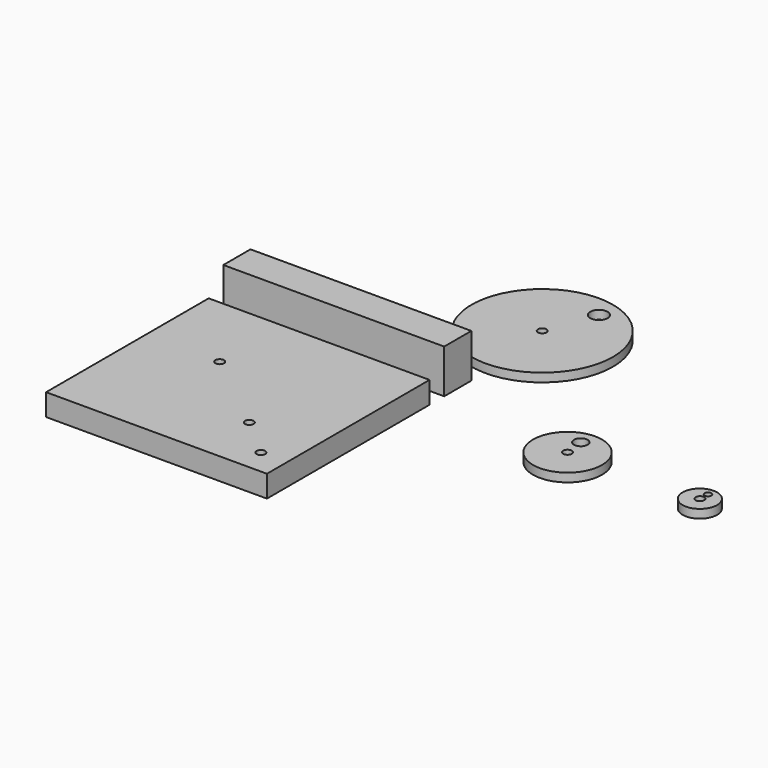
from build123d import *

# Parameters (mm, degrees)
F1_R             = 10
F1_R_2           = 1.9724824491
F2_DEPTH         = 2.5
F1_R_3           = 5
F1_R_4           = 0.9790800152
F0_R             = 20.5
F0_R_2           = 2.5126354118
F3_W             = 64.0254840255
F3_H             = 58.9180318639
F4_DEPTH         = 6.35
F3_H_2           = 9.8366048187
F5_DEPTH         = 6.35
F6_D             = 2.5
F8_D             = 2.5
F8_COPIES_COUNT  = 2
F8_COPIES_PITCH  = 30.5
F8_COPIES1_COUNT = 2
F8_COPIES1_PITCH = 45.489759
F10_D            = 2.5
F10_2_D          = 2.5


# Not quite as in the source:
# - a feature of the source that left no trace in its solid (it failed there, or was rolled back) is left out
# - a pattern or mirror of a feature is missing from the dataset's text; its kind, count and spacing are read off the source's solid


with BuildPart() as f2:
    # F1 (on Top) → F2 (new body)
    with BuildSketch(Plane.XY):
        with Locations((-4.1198744439, 6.6673322581)):
            Circle(F1_R)
        with Locations((-4.8270216212, 12.3583702371)):
            Circle(F1_R_2, mode=Mode.SUBTRACT)
    extrude(amount=F2_DEPTH)

    # F10 (through all)
    with Locations(Plane(origin=(0, 0, 0), x_dir=(1, 0, 0), z_dir=(0, 0, -1))):
        with Locations((-4.1198744439, -6.6673322581), (33.4935821593, -7.599897217)):
            Hole(F10_D / 2)


with BuildPart() as f2b:
    # F1 (on Top) → F2, piece 2 (new body)
    with BuildSketch(Plane.XY):
        with Locations((33.4935821593, 7.599897217)):
            Circle(F1_R_3)
        with Locations((33.6022078991, 10.4110669345)):
            Circle(F1_R_4, mode=Mode.SUBTRACT)
    extrude(amount=F2_DEPTH)

    # F10#2 (through all)
    with Locations(Plane(origin=(0, 0, 0), x_dir=(1, 0, 0), z_dir=(0, 0, -1))):
        with Locations((-4.1198744439, -6.6673322581), (33.4935821593, -7.599897217)):
            Hole(F10_2_D / 2)


with BuildPart() as f2c:
    # F0 (on Top) → F2, piece 3 (new body)
    with BuildSketch(Plane.XY):
        with Locations((-45.774448663, 49.5653226972)):
            Circle(F0_R)
        with Locations((-40.6095050275, 63.6612325907)):
            Circle(F0_R_2, mode=Mode.SUBTRACT)
    extrude(amount=F2_DEPTH)

    # F6 (through all)
    with Locations(Plane(origin=(0, 0, 0), x_dir=(1, 0, 0), z_dir=(0, 0, -1))):
        with Locations((-45.774448663, -49.5653226972)):
            Hole(F6_D / 2)


with BuildPart() as f4:
    # F3 (on Top) → F4 (new body)
    with BuildSketch(Plane.XY):
        with Locations((-78.0650638044, -20.3869701363)):
            Rectangle(F3_W, F3_H)
    extrude(amount=F4_DEPTH)

    # F8 (through all)
    with Locations(Plane.XY.offset(6.35)):
        with Locations((-88.7101224427, -13.6320184063)):
            f8 = Hole(F8_D / 2)

    # F8_copies: F8 ×2
    with Locations(*[Vector(0.7808687891, -0.6246950729, 0) * (i * F8_COPIES_PITCH) for i in range(1, F8_COPIES_COUNT)]):
        add(f8, mode=Mode.SUBTRACT)

    # F8_copies1: F8 ×2
    with Locations(*[Vector(0.7714882729, -0.636243542, 0) * (i * F8_COPIES1_PITCH) for i in range(1, F8_COPIES1_COUNT)]):
        add(f8, mode=Mode.SUBTRACT)


with BuildPart() as f4b:
    # F3 (on Top) → F4, piece 2 (new body)
    with BuildSketch(Plane.XY):
        with Locations((-78.0650638044, 19.3000948057)):
            Rectangle(F3_W, F3_H_2)
    extrude(amount=F4_DEPTH)

    # F5 (add): a face of the model
    f5_faces = [f4b.faces().sort_by_distance(p)[0] for p in [
        (-78.0650638044, 19.3000948057, 6.35),
    ]]
    extrude(f5_faces, amount=F5_DEPTH)


solid = Compound([f2.part, f2b.part, f2c.part, f4.part, f4b.part])
